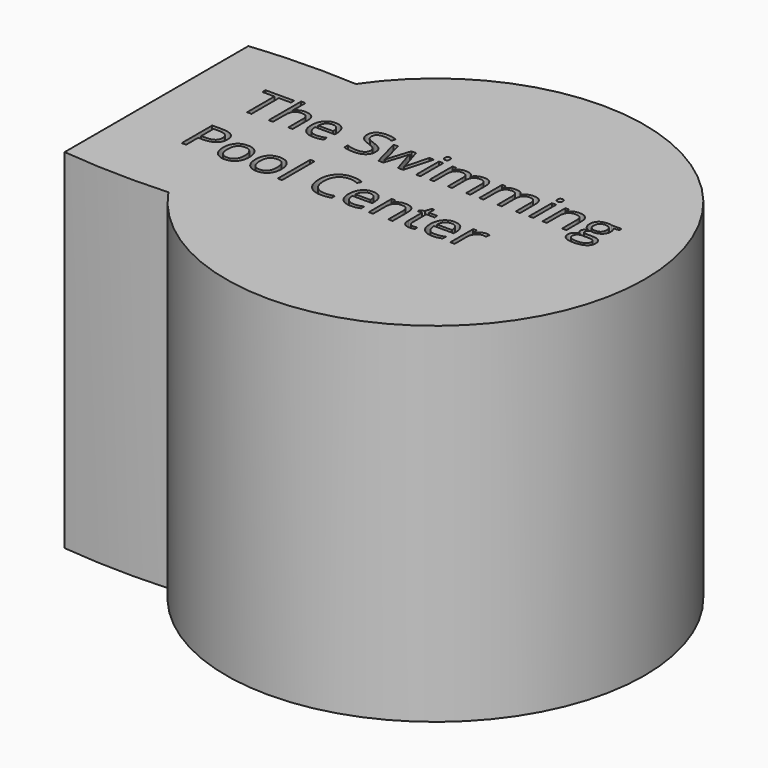
from build123d import *

# Parameters (mm, degrees)
F0_R         = 38.1
F1_DEPTH     = 63.5
F3_DEPTH     = 63.5
F4_W         = 42.6510739346
F4_H         = 45.9493876212
F5_DEPTH     = 38.1
F7_DEPTH     = 59.7
F9_DEPTH     = 126
F8_TEXT_SIZE = 9.7222222222
F10_DEPTH    = 25


# Not quite as in the source:
# - Text() gives the source's letters only with a copy of the font that has no kerning and outlines rounded to 1/6400 em; it was checked with that copy


with BuildPart() as f1:
    # F0 (on Top) → F1 (new body)
    with BuildSketch(Plane.XY):
        Circle(F0_R)
    extrude(amount=F1_DEPTH)

    # F2 (on Top) → F3 (join)
    with BuildSketch(Plane.XY):
        with BuildLine():
            add(Edge.make_bspline(
                [(-89.2776555002, 0), (-89.2776555002, -37.3146463802), (-13.0776555002, -18.6573231901), (63.1223444998, 0), (-13.0776555002, 18.6573231901), (-89.2776555002, 37.3146463802), (-89.2776555002, 0)],
                knots=[0, 0, 0, 2.0943951024, 2.0943951024, 4.1887902048, 4.1887902048, 6.2831853072, 6.2831853072, 6.2831853072], degree=2, weights=[1, 0.5, 1, 0.5, 1, 0.5, 1]))
        make_face()
    extrude(amount=F3_DEPTH)

    # F4 (on Top) → F5 (cut)
    with BuildSketch(Plane.XY):
        with Locations((-72.1255369673, 0.3977268934)):
            Rectangle(F4_W, F4_H)
    extrude(amount=F5_DEPTH, mode=Mode.SUBTRACT)

    # F6 (on Top) → F7 (cut)
    with BuildSketch(Plane.XY):
        with BuildLine():
            ThreePointArc((-29.4796385567, -18.7271603712), (-34.925, 0), (-29.4796385567, 18.7271603712))
            add(Edge.make_bspline(
                [(-29.4796385567, 18.7271603712), (-85.4910984635, 22.6604054842), (-85.4910984635, 0)],
                knots=[4.5379319192, 4.5379319192, 4.5379319192, 6.2831853072, 6.2831853072, 6.2831853072], degree=2, weights=[1, 0.6428166668, 1]))
            add(Edge.make_bspline(
                [(-85.4910984635, 0), (-85.4910984635, -22.6604054842), (-29.4796385567, -18.7271603712)],
                knots=[0, 0, 0, 1.7452533879, 1.7452533879, 1.7452533879], degree=2, weights=[1, 0.6428166668, 1]))
        make_face()
        with BuildLine():
            add(Edge.make_bspline(
                [(-29.4796385567, -18.7271603712), (9.9634453654, -15.9573822341), (9.9634453654, 0), (9.9634453654, 15.9573822341), (-29.4796385567, 18.7271603712)],
                knots=[1.7452533879, 1.7452533879, 1.7452533879, 3.1415926536, 3.1415926536, 4.5379319192, 4.5379319192, 4.5379319192], degree=2, weights=[1, 0.7660200603, 1, 0.7660200603, 1]))
            ThreePointArc((-29.4796385567, 18.7271603712), (-34.925, 0), (-29.4796385567, -18.7271603712))
        make_face()
        with BuildLine():
            ThreePointArc((-29.4796385567, -18.7271603712), (9.7513908856, -33.5360403267), (34.925, 0))
            ThreePointArc((34.925, 0), (9.7513908856, 33.5360403267), (-29.4796385567, 18.7271603712))
            add(Edge.make_bspline(
                [(-29.4796385567, -18.7271603712), (9.9634453654, -15.9573822341), (9.9634453654, 0), (9.9634453654, 15.9573822341), (-29.4796385567, 18.7271603712)],
                knots=[1.7452533879, 1.7452533879, 1.7452533879, 3.1415926536, 3.1415926536, 4.5379319192, 4.5379319192, 4.5379319192], degree=2, weights=[1, 0.7660200603, 1, 0.7660200603, 1]))
        make_face()
    extrude(amount=F7_DEPTH, mode=Mode.SUBTRACT)

    # F4 (on Top) → F9 (cut)
    with BuildSketch(Plane.XY):
        with Locations((-72.1255369673, 0.3977268934)):
            Rectangle(F4_W, F4_H)
    extrude(amount=F9_DEPTH, mode=Mode.SUBTRACT)

    # F8 (on face) → F10 (cut)
    with BuildSketch(Plane.XY.offset(63.5)):
        with Locations((-40.4867779011, 4.8889535827)):
            Text('The Swimming', F8_TEXT_SIZE, font='Open Sans', text_align=(TextAlign.LEFT, TextAlign.BOTTOM))
        with Locations((-40.4867779011, -8.3332686395)):
            Text('Pool Center', F8_TEXT_SIZE, font='Open Sans', text_align=(TextAlign.LEFT, TextAlign.BOTTOM))
    extrude(amount=-F10_DEPTH, mode=Mode.SUBTRACT)


solid = f1.part
